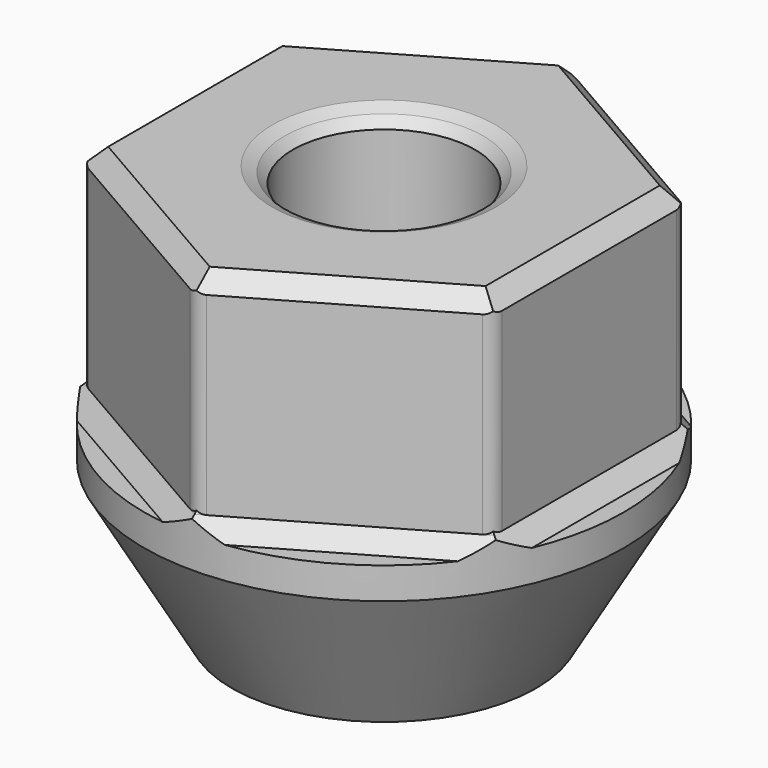
from build123d import *

# Parameters (mm, degrees)
F1_DEPTH       = 19
F2_D           = 8.4328
F2_CSINK_D     = 9.652
F2_CSINK_ANGLE = 82
F3_R           = 11.1125
F3_R_2         = 4.2164
F4_DEPTH       = 8.5
F5_SIZE2       = 7.039054482
F5_SIZE        = 4.064
F6_T1_DEPTH    = 14.8888999883
F6_T3_DEPTH    = 14.8888999883
F6_T5_DEPTH    = 14.8888999883
F6_T7_DEPTH    = 14.8888999883
F6_T9_DEPTH    = 14.8888999883
F7_T4_DEPTH    = 14.8888999883
F7_S5_R        = 11.1125
F7_T6_DEPTH    = 9
F7_T12_DEPTH   = 14.8888999883
F7_S13_R       = 11.1125
F7_T14_DEPTH   = 9
F7_T20_DEPTH   = 14.8888999883
F7_S21_R       = 11.1125
F7_T22_DEPTH   = 9
F7_T28_DEPTH   = 14.8888999883
F7_S29_R       = 11.1125
F7_T30_DEPTH   = 9
F7_T36_DEPTH   = 14.8888999883
F7_S37_R       = 11.1125
F7_T38_DEPTH   = 9
F7_T44_DEPTH   = 14.8888999883
F7_S45_R       = 11.1125
F7_T46_DEPTH   = 9
F7_T53_DEPTH   = 14.8888999883
F7_S54_R       = 11.1125
F7_T55_DEPTH   = 9
F7_T59_DEPTH   = 14.8888999883
F7_S60_R       = 11.1125
F7_T61_DEPTH   = 9
F7_T68_DEPTH   = 14.8888999883
F7_S69_R       = 11.1125
F7_T70_DEPTH   = 9
F7_T74_DEPTH   = 14.8888999883
F7_S75_R       = 11.1125
F7_T76_DEPTH   = 9
F7_T83_DEPTH   = 14.8888999883
F7_S84_R       = 11.1125
F7_T85_DEPTH   = 9
F7_T89_DEPTH   = 14.8888999883
F7_S90_R       = 11.1125
F7_T91_DEPTH   = 9
F7_T98_DEPTH   = 14.8888999883
F7_S99_R       = 11.1125
F7_T100_DEPTH  = 9
F7_T104_DEPTH  = 14.8888999883
F7_S105_R      = 11.1125
F7_T106_DEPTH  = 9
F7_T113_DEPTH  = 14.8888999883
F7_S114_R      = 11.1125
F7_T115_DEPTH  = 9
F7_T119_DEPTH  = 14.8888999883
F7_S120_R      = 11.1125
F7_T121_DEPTH  = 9
F7_T128_DEPTH  = 14.8888999883
F7_S129_R      = 11.1125
F7_T130_DEPTH  = 9
F7_T134_DEPTH  = 14.8888999883
F7_S135_R      = 11.1125
F7_T136_DEPTH  = 9
F8_T4_DEPTH    = 11.1757045256
F8_T10_DEPTH   = 11.1757045256
F8_T16_DEPTH   = 11.1757045256
F8_T22_DEPTH   = 11.1757045256
F8_T28_DEPTH   = 11.1757045256
F8_T34_DEPTH   = 11.1757045256
F8_T40_DEPTH   = 11.1757045256
F8_T46_DEPTH   = 11.1757045256
F8_T52_DEPTH   = 11.1757045256
F8_T58_DEPTH   = 11.1757045256
F8_T64_DEPTH   = 11.1757045256
F8_T70_DEPTH   = 11.1757045256
F8_T76_DEPTH   = 11.1757045256
F8_T82_DEPTH   = 11.1757045256
F8_T88_DEPTH   = 11.1757045256
F8_T94_DEPTH   = 11.1757045256
F8_T100_DEPTH  = 11.1757045256
F8_T106_DEPTH  = 11.1757045256


# Not quite as in the source:
# - a fillet or chamfer that OpenCascade refuses, or shapes differently, is made with other operations: its cross-section is extruded or revolved along the edge and cut away or added


with BuildPart() as f1:
    # F0 (on Top) → F1 (new body)
    with BuildSketch(Plane.XY):
        Polygon((9.5, -5.4848275573), (9.5, 5.4848275573), (0, 10.9696551146), (-9.5, 5.4848275573), (-9.5, -5.4848275573), (0, -10.9696551146), align=None)
    extrude(amount=-F1_DEPTH)

    # F2 (through all)
    with Locations(Plane.XY):
        with Locations((0, 0)):
            CounterSinkHole(F2_D / 2, F2_CSINK_D / 2, counter_sink_angle=F2_CSINK_ANGLE)

    # F3 (on face) → F4 (join)
    with BuildSketch(Plane(origin=(0, 0, -19), x_dir=(1, 0, 0), z_dir=(0, 0, -1))):
        Circle(F3_R)
        Circle(F3_R_2, mode=Mode.SUBTRACT)
    extrude(amount=-F4_DEPTH)

    # F5
    f5_edges = [f1.edges().sort_by_distance(p)[0] for p in [
        (-11.1125, 0, -19),
    ]]
    f5_side = f1.faces().sort_by_distance((-10.798191, 0, -19))[0]
    chamfer(f5_edges, length=F5_SIZE, length2=F5_SIZE2, reference=f5_side)

    # F6: chamfer of 0.762 on 7 edges, made by hand

    # F6_s2 → F6_t1 (cut)
    with BuildSketch(Plane.XZ.offset(-7.4444499941)):
        Polygon((9.5, -0.762), (8.738, 0), (9.5, 0), align=None)
        Polygon((-9.5, -0.762), (-8.738, 0), (-9.5, 0), align=None)
    extrude(amount=F6_T1_DEPTH, mode=Mode.SUBTRACT)

    # F6_s4 → F6_t3 (cut)
    with BuildSketch(Plane(origin=(-6.4470828121, -3.7222249971, 0), x_dir=(0, 0, 1), z_dir=(0.8660254038, 0.5, 0))):
        Polygon((-0.762, 9.5), (0, 8.738), (0, 9.5), align=None)
    extrude(amount=F6_T3_DEPTH, mode=Mode.SUBTRACT)

    # F6_s6 → F6_t5 (cut)
    with BuildSketch(Plane(origin=(6.4470828121, -3.7222249971, 0), x_dir=(0, 0, 1), z_dir=(-0.8660254038, 0.5, 0))):
        Polygon((-0.762, 9.5), (0, 8.738), (0, 9.5), align=None)
    extrude(amount=F6_T5_DEPTH, mode=Mode.SUBTRACT)

    # F6_s8 → F6_t7 (cut)
    with BuildSketch(Plane(origin=(-6.4470828121, 3.7222249971, 0), x_dir=(0, 0, 1), z_dir=(0.8660254038, -0.5, 0))):
        Polygon((-0.762, 9.5), (0, 8.738), (0, 9.5), align=None)
    extrude(amount=F6_T7_DEPTH, mode=Mode.SUBTRACT)

    # F6_s10 → F6_t9 (cut)
    with BuildSketch(Plane(origin=(6.4470828121, 3.7222249971, 0), x_dir=(0, 0, 1), z_dir=(-0.8660254038, -0.5, 0))):
        Polygon((-0.762, 9.5), (0, 8.738), (0, 9.5), align=None)
    extrude(amount=F6_T9_DEPTH, mode=Mode.SUBTRACT)

    # F6_s11 → F6_t12 (revolve, cut)
    with BuildSketch(Plane.XZ):
        Polygon((5.1727200241, 0), (4.5972787828, -0.2624888611), (4.8251319511, 0), align=None)
    revolve(axis=Axis((0, 0, 0), (0, 0, 1)), mode=Mode.SUBTRACT)

    # F7: chamfer of 0.762 on 6 edges, made by hand


with BuildPart() as f7_tool2:
    # F7_s3 → F7_t4 (new body)
    with BuildSketch(Plane(origin=(-6.4470828121, 3.7222249971, 0), x_dir=(0, 0, 1), z_dir=(0.8660254038, -0.5, 0))):
        Polygon((-10.5, 10.262), (-9.738, 9.5), (-10.5, 9.5), align=None)
    extrude(amount=F7_T4_DEPTH)

    # F7_s5 → F7_t6 (intersect, symmetric)
    with BuildSketch(Plane.XY.offset(-10.1)):
        Circle(F7_S5_R)
    extrude(amount=F7_T6_DEPTH, both=True, mode=Mode.INTERSECT)

    split(bisect_by=Plane(origin=(4.75, -8.227241336, 0), x_dir=(0, 0, 1), z_dir=(-0.5, 0.8660254038, 0)), keep=Keep.TOP)

    split(bisect_by=Plane.YZ.offset(-9.5), keep=Keep.TOP)


with BuildPart() as f1_1:
    add(f1.part)

    # F7_t1: union F7_tool2
    add(f7_tool2.part)


with BuildPart() as f7_tool10:
    # F7_s11 → F7_t12 (new body)
    with BuildSketch(Plane(origin=(-6.4470828121, -3.7222249971, 0), x_dir=(0, 0, 1), z_dir=(0.8660254038, 0.5, 0))):
        Polygon((-10.5, 10.262), (-9.738, 9.5), (-10.5, 9.5), align=None)
    extrude(amount=F7_T12_DEPTH)

    # F7_s13 → F7_t14 (intersect, symmetric)
    with BuildSketch(Plane.XY.offset(-10.1)):
        Circle(F7_S13_R)
    extrude(amount=F7_T14_DEPTH, both=True, mode=Mode.INTERSECT)

    split(bisect_by=Plane.YZ.offset(9.5), keep=Keep.BOTTOM)

    split(bisect_by=Plane(origin=(-4.75, -8.227241336, 0), x_dir=(0, 0, 1), z_dir=(0.5, 0.8660254038, 0)), keep=Keep.TOP)


with BuildPart() as f1_2:
    add(f1_1.part)

    # F7_t9: union F7_tool10
    add(f7_tool10.part)


with BuildPart() as f7_tool18:
    # F7_s19 → F7_t20 (new body)
    with BuildSketch(Plane.XZ.offset(7.4444499941)):
        Polygon((10.262, -10.5), (9.5, -9.738), (9.5, -10.5), align=None)
    extrude(amount=-F7_T20_DEPTH)

    # F7_s21 → F7_t22 (intersect, symmetric)
    with BuildSketch(Plane.XY.offset(-10.1)):
        Circle(F7_S21_R)
    extrude(amount=F7_T22_DEPTH, both=True, mode=Mode.INTERSECT)

    split(bisect_by=Plane(origin=(4.75, -8.227241336, 0), x_dir=(0, 0, 1), z_dir=(-0.5, 0.8660254038, 0)), keep=Keep.TOP)

    split(bisect_by=Plane(origin=(4.75, 8.227241336, 0), x_dir=(0, 0, 1), z_dir=(-0.5, -0.8660254038, 0)), keep=Keep.TOP)


with BuildPart() as f1_3:
    add(f1_2.part)

    # F7_t17: union F7_tool18
    add(f7_tool18.part)


with BuildPart() as f7_tool26:
    # F7_s27 → F7_t28 (new body)
    with BuildSketch(Plane(origin=(6.4470828121, -3.7222249971, 0), x_dir=(0, 0, 1), z_dir=(-0.8660254038, 0.5, 0))):
        Polygon((-10.5, 10.262), (-9.738, 9.5), (-10.5, 9.5), align=None)
    extrude(amount=F7_T28_DEPTH)

    # F7_s29 → F7_t30 (intersect, symmetric)
    with BuildSketch(Plane.XY.offset(-10.1)):
        Circle(F7_S29_R)
    extrude(amount=F7_T30_DEPTH, both=True, mode=Mode.INTERSECT)

    split(bisect_by=Plane(origin=(-4.75, 8.227241336, 0), x_dir=(0, 0, 1), z_dir=(0.5, -0.8660254038, 0)), keep=Keep.TOP)

    split(bisect_by=Plane.YZ.offset(9.5), keep=Keep.BOTTOM)


with BuildPart() as f1_4:
    add(f1_3.part)

    # F7_t25: union F7_tool26
    add(f7_tool26.part)


with BuildPart() as f7_tool34:
    # F7_s35 → F7_t36 (new body)
    with BuildSketch(Plane(origin=(6.4470828121, 3.7222249971, 0), x_dir=(0, 0, 1), z_dir=(-0.8660254038, -0.5, 0))):
        Polygon((-10.5, 10.262), (-9.738, 9.5), (-10.5, 9.5), align=None)
    extrude(amount=F7_T36_DEPTH)

    # F7_s37 → F7_t38 (intersect, symmetric)
    with BuildSketch(Plane.XY.offset(-10.1)):
        Circle(F7_S37_R)
    extrude(amount=F7_T38_DEPTH, both=True, mode=Mode.INTERSECT)

    split(bisect_by=Plane.YZ.offset(-9.5), keep=Keep.TOP)

    split(bisect_by=Plane(origin=(4.75, 8.227241336, 0), x_dir=(0, 0, 1), z_dir=(-0.5, -0.8660254038, 0)), keep=Keep.TOP)


with BuildPart() as f1_5:
    add(f1_4.part)

    # F7_t33: union F7_tool34
    add(f7_tool34.part)


with BuildPart() as f7_tool42:
    # F7_s43 → F7_t44 (new body)
    with BuildSketch(Plane.XZ.offset(-7.4444499941)):
        Polygon((-10.262, -10.5), (-9.5, -9.738), (-9.5, -10.5), align=None)
    extrude(amount=F7_T44_DEPTH)

    # F7_s45 → F7_t46 (intersect, symmetric)
    with BuildSketch(Plane.XY.offset(-10.1)):
        Circle(F7_S45_R)
    extrude(amount=F7_T46_DEPTH, both=True, mode=Mode.INTERSECT)

    split(bisect_by=Plane(origin=(-4.75, -8.227241336, 0), x_dir=(0, 0, 1), z_dir=(0.5, 0.8660254038, 0)), keep=Keep.TOP)

    split(bisect_by=Plane(origin=(-4.75, 8.227241336, 0), x_dir=(0, 0, 1), z_dir=(0.5, -0.8660254038, 0)), keep=Keep.TOP)


with BuildPart() as f1_6:
    add(f1_5.part)

    # F7_t41: union F7_tool42
    add(f7_tool42.part)


with BuildPart() as f7_tool51:
    # F7_s52 → F7_t53 (new body)
    with BuildSketch(Plane(origin=(-6.4470828121, 3.7222249971, 0), x_dir=(0, 0, 1), z_dir=(0.8660254038, -0.5, 0))):
        Polygon((-10.5, 10.262), (-9.738, 9.5), (-10.5, 9.5), align=None)
    extrude(amount=F7_T53_DEPTH)

    # F7_s54 → F7_t55 (intersect, symmetric)
    with BuildSketch(Plane.XY.offset(-10.1)):
        Circle(F7_S54_R)
    extrude(amount=F7_T55_DEPTH, both=True, mode=Mode.INTERSECT)

    split(bisect_by=Plane.YZ.offset(-9.5), keep=Keep.BOTTOM)


with BuildPart() as f7_tool57:
    # F7_s58 → F7_t59 (new body)
    with BuildSketch(Plane.XZ.offset(-7.4444499941)):
        Polygon((-10.262, -10.5), (-9.5, -9.738), (-9.5, -10.5), align=None)
    extrude(amount=F7_T59_DEPTH)

    # F7_s60 → F7_t61 (intersect, symmetric)
    with BuildSketch(Plane.XY.offset(-10.1)):
        Circle(F7_S60_R)
    extrude(amount=F7_T61_DEPTH, both=True, mode=Mode.INTERSECT)

    split(bisect_by=Plane(origin=(-4.75, -8.227241336, 0), x_dir=(0, 0, 1), z_dir=(-0.5, -0.8660254038, 0)), keep=Keep.TOP)


with BuildPart() as f7_tool51_1:
    add(f7_tool51.part)

    # F7_t63: intersect F7_tool57
    add(f7_tool57.part, mode=Mode.INTERSECT)


with BuildPart() as f1_7:
    add(f1_6.part)

    # F7_t49: union F7_tool51
    add(f7_tool51_1.part)


with BuildPart() as f7_tool66:
    # F7_s67 → F7_t68 (new body)
    with BuildSketch(Plane(origin=(-6.4470828121, -3.7222249971, 0), x_dir=(0, 0, 1), z_dir=(0.8660254038, 0.5, 0))):
        Polygon((-10.5, 10.262), (-9.738, 9.5), (-10.5, 9.5), align=None)
    extrude(amount=F7_T68_DEPTH)

    # F7_s69 → F7_t70 (intersect, symmetric)
    with BuildSketch(Plane.XY.offset(-10.1)):
        Circle(F7_S69_R)
    extrude(amount=F7_T70_DEPTH, both=True, mode=Mode.INTERSECT)

    split(bisect_by=Plane(origin=(-4.75, -8.227241336, 0), x_dir=(0, 0, 1), z_dir=(-0.5, -0.8660254038, 0)), keep=Keep.TOP)


with BuildPart() as f7_tool72:
    # F7_s73 → F7_t74 (new body)
    with BuildSketch(Plane(origin=(-6.4470828121, 3.7222249971, 0), x_dir=(0, 0, 1), z_dir=(0.8660254038, -0.5, 0))):
        Polygon((-10.5, 10.262), (-9.738, 9.5), (-10.5, 9.5), align=None)
    extrude(amount=F7_T74_DEPTH)

    # F7_s75 → F7_t76 (intersect, symmetric)
    with BuildSketch(Plane.XY.offset(-10.1)):
        Circle(F7_S75_R)
    extrude(amount=F7_T76_DEPTH, both=True, mode=Mode.INTERSECT)

    split(bisect_by=Plane(origin=(4.75, -8.227241336, 0), x_dir=(0, 0, 1), z_dir=(0.5, -0.8660254038, 0)), keep=Keep.TOP)


with BuildPart() as f7_tool66_1:
    add(f7_tool66.part)

    # F7_t78: intersect F7_tool72
    add(f7_tool72.part, mode=Mode.INTERSECT)


with BuildPart() as f1_8:
    add(f1_7.part)

    # F7_t64: union F7_tool66
    add(f7_tool66_1.part)


with BuildPart() as f7_tool81:
    # F7_s82 → F7_t83 (new body)
    with BuildSketch(Plane(origin=(-6.4470828121, -3.7222249971, 0), x_dir=(0, 0, 1), z_dir=(0.8660254038, 0.5, 0))):
        Polygon((-10.5, 10.262), (-9.738, 9.5), (-10.5, 9.5), align=None)
    extrude(amount=F7_T83_DEPTH)

    # F7_s84 → F7_t85 (intersect, symmetric)
    with BuildSketch(Plane.XY.offset(-10.1)):
        Circle(F7_S84_R)
    extrude(amount=F7_T85_DEPTH, both=True, mode=Mode.INTERSECT)

    split(bisect_by=Plane.YZ.offset(9.5), keep=Keep.TOP)


with BuildPart() as f7_tool87:
    # F7_s88 → F7_t89 (new body)
    with BuildSketch(Plane.XZ.offset(7.4444499941)):
        Polygon((10.262, -10.5), (9.5, -9.738), (9.5, -10.5), align=None)
    extrude(amount=-F7_T89_DEPTH)

    # F7_s90 → F7_t91 (intersect, symmetric)
    with BuildSketch(Plane.XY.offset(-10.1)):
        Circle(F7_S90_R)
    extrude(amount=F7_T91_DEPTH, both=True, mode=Mode.INTERSECT)

    split(bisect_by=Plane(origin=(4.75, -8.227241336, 0), x_dir=(0, 0, 1), z_dir=(0.5, -0.8660254038, 0)), keep=Keep.TOP)


with BuildPart() as f7_tool81_1:
    add(f7_tool81.part)

    # F7_t93: intersect F7_tool87
    add(f7_tool87.part, mode=Mode.INTERSECT)


with BuildPart() as f1_9:
    add(f1_8.part)

    # F7_t79: union F7_tool81
    add(f7_tool81_1.part)


with BuildPart() as f7_tool96:
    # F7_s97 → F7_t98 (new body)
    with BuildSketch(Plane(origin=(6.4470828121, -3.7222249971, 0), x_dir=(0, 0, 1), z_dir=(-0.8660254038, 0.5, 0))):
        Polygon((-10.5, 10.262), (-9.738, 9.5), (-10.5, 9.5), align=None)
    extrude(amount=F7_T98_DEPTH)

    # F7_s99 → F7_t100 (intersect, symmetric)
    with BuildSketch(Plane.XY.offset(-10.1)):
        Circle(F7_S99_R)
    extrude(amount=F7_T100_DEPTH, both=True, mode=Mode.INTERSECT)

    split(bisect_by=Plane.YZ.offset(9.5), keep=Keep.TOP)


with BuildPart() as f7_tool102:
    # F7_s103 → F7_t104 (new body)
    with BuildSketch(Plane.XZ.offset(7.4444499941)):
        Polygon((10.262, -10.5), (9.5, -9.738), (9.5, -10.5), align=None)
    extrude(amount=-F7_T104_DEPTH)

    # F7_s105 → F7_t106 (intersect, symmetric)
    with BuildSketch(Plane.XY.offset(-10.1)):
        Circle(F7_S105_R)
    extrude(amount=F7_T106_DEPTH, both=True, mode=Mode.INTERSECT)

    split(bisect_by=Plane(origin=(4.75, 8.227241336, 0), x_dir=(0, 0, 1), z_dir=(0.5, 0.8660254038, 0)), keep=Keep.TOP)


with BuildPart() as f7_tool96_1:
    add(f7_tool96.part)

    # F7_t108: intersect F7_tool102
    add(f7_tool102.part, mode=Mode.INTERSECT)


with BuildPart() as f1_10:
    add(f1_9.part)

    # F7_t94: union F7_tool96
    add(f7_tool96_1.part)


with BuildPart() as f7_tool111:
    # F7_s112 → F7_t113 (new body)
    with BuildSketch(Plane(origin=(6.4470828121, 3.7222249971, 0), x_dir=(0, 0, 1), z_dir=(-0.8660254038, -0.5, 0))):
        Polygon((-10.5, 10.262), (-9.738, 9.5), (-10.5, 9.5), align=None)
    extrude(amount=F7_T113_DEPTH)

    # F7_s114 → F7_t115 (intersect, symmetric)
    with BuildSketch(Plane.XY.offset(-10.1)):
        Circle(F7_S114_R)
    extrude(amount=F7_T115_DEPTH, both=True, mode=Mode.INTERSECT)

    split(bisect_by=Plane(origin=(4.75, 8.227241336, 0), x_dir=(0, 0, 1), z_dir=(0.5, 0.8660254038, 0)), keep=Keep.TOP)


with BuildPart() as f7_tool117:
    # F7_s118 → F7_t119 (new body)
    with BuildSketch(Plane(origin=(6.4470828121, -3.7222249971, 0), x_dir=(0, 0, 1), z_dir=(-0.8660254038, 0.5, 0))):
        Polygon((-10.5, 10.262), (-9.738, 9.5), (-10.5, 9.5), align=None)
    extrude(amount=F7_T119_DEPTH)

    # F7_s120 → F7_t121 (intersect, symmetric)
    with BuildSketch(Plane.XY.offset(-10.1)):
        Circle(F7_S120_R)
    extrude(amount=F7_T121_DEPTH, both=True, mode=Mode.INTERSECT)

    split(bisect_by=Plane(origin=(-4.75, 8.227241336, 0), x_dir=(0, 0, 1), z_dir=(-0.5, 0.8660254038, 0)), keep=Keep.TOP)


with BuildPart() as f7_tool111_1:
    add(f7_tool111.part)

    # F7_t123: intersect F7_tool117
    add(f7_tool117.part, mode=Mode.INTERSECT)


with BuildPart() as f1_11:
    add(f1_10.part)

    # F7_t109: union F7_tool111
    add(f7_tool111_1.part)


with BuildPart() as f7_tool126:
    # F7_s127 → F7_t128 (new body)
    with BuildSketch(Plane.XZ.offset(-7.4444499941)):
        Polygon((-10.262, -10.5), (-9.5, -9.738), (-9.5, -10.5), align=None)
    extrude(amount=F7_T128_DEPTH)

    # F7_s129 → F7_t130 (intersect, symmetric)
    with BuildSketch(Plane.XY.offset(-10.1)):
        Circle(F7_S129_R)
    extrude(amount=F7_T130_DEPTH, both=True, mode=Mode.INTERSECT)

    split(bisect_by=Plane(origin=(-4.75, 8.227241336, 0), x_dir=(0, 0, 1), z_dir=(-0.5, 0.8660254038, 0)), keep=Keep.TOP)


with BuildPart() as f7_tool132:
    # F7_s133 → F7_t134 (new body)
    with BuildSketch(Plane(origin=(6.4470828121, 3.7222249971, 0), x_dir=(0, 0, 1), z_dir=(-0.8660254038, -0.5, 0))):
        Polygon((-10.5, 10.262), (-9.738, 9.5), (-10.5, 9.5), align=None)
    extrude(amount=F7_T134_DEPTH)

    # F7_s135 → F7_t136 (intersect, symmetric)
    with BuildSketch(Plane.XY.offset(-10.1)):
        Circle(F7_S135_R)
    extrude(amount=F7_T136_DEPTH, both=True, mode=Mode.INTERSECT)

    split(bisect_by=Plane.YZ.offset(-9.5), keep=Keep.BOTTOM)


with BuildPart() as f7_tool126_1:
    add(f7_tool126.part)

    # F7_t138: intersect F7_tool132
    add(f7_tool132.part, mode=Mode.INTERSECT)


with BuildPart() as f1_12:
    add(f1_11.part)

    # F7_t124: union F7_tool126
    add(f7_tool126_1.part)

    # F8: fillet of radius 0.762 on 6 edges, made by hand


with BuildPart() as f8_tool2:
    # F8_s3 → F8_t4 (new body)
    with BuildSketch(Plane.XY.offset(0.3378522628)):
        with BuildLine():
            ThreePointArc((9.5, -5.0448866522), (9.3979113577, -5.4258866522), (9.119, -5.7047980099))
            Line((9.119, -5.7047980099), (9.5, -5.4848275573))
            Line((9.5, -5.4848275573), (9.5, -5.0448866522))
        make_face()
    extrude(amount=-F8_T4_DEPTH)

    split(bisect_by=Plane(origin=(-0.119, 0, -0.119), x_dir=(0, 1, 0), z_dir=(0.7071067812, 0, 0.7071067812)), keep=Keep.TOP)

    split(bisect_by=Plane(origin=(-0.0595, 0.1030570231, -0.119), x_dir=(0.8660254038, 0.5, 0), z_dir=(0.3535533906, -0.6123724357, 0.7071067812)), keep=Keep.TOP)


with BuildPart() as f1_13:
    add(f1_12.part)

    # F8_t1: cut F8_tool2
    add(f8_tool2.part, mode=Mode.SUBTRACT)


with BuildPart() as f8_tool8:
    # F8_s9 → F8_t10 (new body)
    with BuildSketch(Plane.XY.offset(0.3378522628)):
        with BuildLine():
            ThreePointArc((9.5, -5.0448866522), (9.3979113577, -5.4258866522), (9.119, -5.7047980099))
            Line((9.119, -5.7047980099), (9.5, -5.4848275573))
            Line((9.5, -5.4848275573), (9.5, -5.0448866522))
        make_face()
    extrude(amount=-F8_T10_DEPTH)

    split(bisect_by=Plane(origin=(-0.119, 0, -0.119), x_dir=(0, 1, 0), z_dir=(-0.7071067812, 0, -0.7071067812)), keep=Keep.TOP)

    split(bisect_by=Plane(origin=(-0.0595, 0.1030570231, -0.119), x_dir=(0.8660254038, 0.5, 0), z_dir=(0.3535533906, -0.6123724357, 0.7071067812)), keep=Keep.TOP)


with BuildPart() as f1_14:
    add(f1_13.part)

    # F8_t7: cut F8_tool8
    add(f8_tool8.part, mode=Mode.SUBTRACT)


with BuildPart() as f8_tool14:
    # F8_s15 → F8_t16 (new body)
    with BuildSketch(Plane.XY.offset(0.3378522628)):
        with BuildLine():
            ThreePointArc((9.5, -5.0448866522), (9.3979113577, -5.4258866522), (9.119, -5.7047980099))
            Line((9.119, -5.7047980099), (9.5, -5.4848275573))
            Line((9.5, -5.4848275573), (9.5, -5.0448866522))
        make_face()
    extrude(amount=-F8_T16_DEPTH)

    split(bisect_by=Plane(origin=(-0.119, 0, -0.119), x_dir=(0, 1, 0), z_dir=(0.7071067812, 0, 0.7071067812)), keep=Keep.TOP)

    split(bisect_by=Plane(origin=(-0.0595, 0.1030570231, -0.119), x_dir=(-0.8660254038, -0.5, 0), z_dir=(-0.3535533906, 0.6123724357, -0.7071067812)), keep=Keep.TOP)


with BuildPart() as f1_15:
    add(f1_14.part)

    # F8_t13: cut F8_tool14
    add(f8_tool14.part, mode=Mode.SUBTRACT)


with BuildPart() as f8_tool20:
    # F8_s21 → F8_t22 (new body)
    with BuildSketch(Plane.XY.offset(0.3378522628)):
        with BuildLine():
            ThreePointArc((-0.381, -10.749684662), (0, -10.8517733044), (0.381, -10.749684662))
            Line((0.381, -10.749684662), (0, -10.9696551146))
            Line((0, -10.9696551146), (-0.381, -10.749684662))
        make_face()
    extrude(amount=-F8_T22_DEPTH)

    split(bisect_by=Plane(origin=(0.0595, 0.1030570231, -0.119), x_dir=(0.8660254038, -0.5, 0), z_dir=(-0.3535533906, -0.6123724357, 0.7071067812)), keep=Keep.TOP)

    split(bisect_by=Plane(origin=(-0.0595, 0.1030570231, -0.119), x_dir=(0.8660254038, 0.5, 0), z_dir=(0.3535533906, -0.6123724357, 0.7071067812)), keep=Keep.TOP)


with BuildPart() as f1_16:
    add(f1_15.part)

    # F8_t19: cut F8_tool20
    add(f8_tool20.part, mode=Mode.SUBTRACT)


with BuildPart() as f8_tool26:
    # F8_s27 → F8_t28 (new body)
    with BuildSketch(Plane.XY.offset(0.3378522628)):
        with BuildLine():
            ThreePointArc((-0.381, -10.749684662), (0, -10.8517733044), (0.381, -10.749684662))
            Line((0.381, -10.749684662), (0, -10.9696551146))
            Line((0, -10.9696551146), (-0.381, -10.749684662))
        make_face()
    extrude(amount=-F8_T28_DEPTH)

    split(bisect_by=Plane(origin=(0.0595, 0.1030570231, -0.119), x_dir=(-0.8660254038, 0.5, 0), z_dir=(0.3535533906, 0.6123724357, -0.7071067812)), keep=Keep.TOP)

    split(bisect_by=Plane(origin=(-0.0595, 0.1030570231, -0.119), x_dir=(0.8660254038, 0.5, 0), z_dir=(0.3535533906, -0.6123724357, 0.7071067812)), keep=Keep.TOP)


with BuildPart() as f1_17:
    add(f1_16.part)

    # F8_t25: cut F8_tool26
    add(f8_tool26.part, mode=Mode.SUBTRACT)


with BuildPart() as f8_tool32:
    # F8_s33 → F8_t34 (new body)
    with BuildSketch(Plane.XY.offset(0.3378522628)):
        with BuildLine():
            ThreePointArc((-0.381, -10.749684662), (0, -10.8517733044), (0.381, -10.749684662))
            Line((0.381, -10.749684662), (0, -10.9696551146))
            Line((0, -10.9696551146), (-0.381, -10.749684662))
        make_face()
    extrude(amount=-F8_T34_DEPTH)

    split(bisect_by=Plane(origin=(0.0595, 0.1030570231, -0.119), x_dir=(0.8660254038, -0.5, 0), z_dir=(-0.3535533906, -0.6123724357, 0.7071067812)), keep=Keep.TOP)

    split(bisect_by=Plane(origin=(-0.0595, 0.1030570231, -0.119), x_dir=(-0.8660254038, -0.5, 0), z_dir=(-0.3535533906, 0.6123724357, -0.7071067812)), keep=Keep.TOP)


with BuildPart() as f1_18:
    add(f1_17.part)

    # F8_t31: cut F8_tool32
    add(f8_tool32.part, mode=Mode.SUBTRACT)


with BuildPart() as f8_tool38:
    # F8_s39 → F8_t40 (new body)
    with BuildSketch(Plane.XY.offset(0.3378522628)):
        with BuildLine():
            ThreePointArc((-9.5, -5.0448866522), (-9.3979113577, -5.4258866522), (-9.119, -5.7047980099))
            Line((-9.119, -5.7047980099), (-9.5, -5.4848275573))
            Line((-9.5, -5.4848275573), (-9.5, -5.0448866522))
        make_face()
    extrude(amount=-F8_T40_DEPTH)

    split(bisect_by=Plane(origin=(0.119, 0, -0.119), x_dir=(0, 1, 0), z_dir=(-0.7071067812, 0, 0.7071067812)), keep=Keep.TOP)

    split(bisect_by=Plane(origin=(0.0595, 0.1030570231, -0.119), x_dir=(0.8660254038, -0.5, 0), z_dir=(-0.3535533906, -0.6123724357, 0.7071067812)), keep=Keep.TOP)


with BuildPart() as f1_19:
    add(f1_18.part)

    # F8_t37: cut F8_tool38
    add(f8_tool38.part, mode=Mode.SUBTRACT)


with BuildPart() as f8_tool44:
    # F8_s45 → F8_t46 (new body)
    with BuildSketch(Plane.XY.offset(0.3378522628)):
        with BuildLine():
            ThreePointArc((-9.5, -5.0448866522), (-9.3979113577, -5.4258866522), (-9.119, -5.7047980099))
            Line((-9.119, -5.7047980099), (-9.5, -5.4848275573))
            Line((-9.5, -5.4848275573), (-9.5, -5.0448866522))
        make_face()
    extrude(amount=-F8_T46_DEPTH)

    split(bisect_by=Plane(origin=(0.119, 0, -0.119), x_dir=(0, 1, 0), z_dir=(0.7071067812, 0, -0.7071067812)), keep=Keep.TOP)

    split(bisect_by=Plane(origin=(0.0595, 0.1030570231, -0.119), x_dir=(0.8660254038, -0.5, 0), z_dir=(-0.3535533906, -0.6123724357, 0.7071067812)), keep=Keep.TOP)


with BuildPart() as f1_20:
    add(f1_19.part)

    # F8_t43: cut F8_tool44
    add(f8_tool44.part, mode=Mode.SUBTRACT)


with BuildPart() as f8_tool50:
    # F8_s51 → F8_t52 (new body)
    with BuildSketch(Plane.XY.offset(0.3378522628)):
        with BuildLine():
            ThreePointArc((-9.5, -5.0448866522), (-9.3979113577, -5.4258866522), (-9.119, -5.7047980099))
            Line((-9.119, -5.7047980099), (-9.5, -5.4848275573))
            Line((-9.5, -5.4848275573), (-9.5, -5.0448866522))
        make_face()
    extrude(amount=-F8_T52_DEPTH)

    split(bisect_by=Plane(origin=(0.119, 0, -0.119), x_dir=(0, 1, 0), z_dir=(-0.7071067812, 0, 0.7071067812)), keep=Keep.TOP)

    split(bisect_by=Plane(origin=(0.0595, 0.1030570231, -0.119), x_dir=(-0.8660254038, 0.5, 0), z_dir=(0.3535533906, 0.6123724357, -0.7071067812)), keep=Keep.TOP)


with BuildPart() as f1_21:
    add(f1_20.part)

    # F8_t49: cut F8_tool50
    add(f8_tool50.part, mode=Mode.SUBTRACT)


with BuildPart() as f8_tool56:
    # F8_s57 → F8_t58 (new body)
    with BuildSketch(Plane.XY.offset(0.3378522628)):
        with BuildLine():
            ThreePointArc((-9.119, 5.7047980099), (-9.3979113577, 5.4258866522), (-9.5, 5.0448866522))
            Line((-9.5, 5.0448866522), (-9.5, 5.4848275573))
            Line((-9.5, 5.4848275573), (-9.119, 5.7047980099))
        make_face()
    extrude(amount=-F8_T58_DEPTH)

    split(bisect_by=Plane(origin=(0.0595, -0.1030570231, -0.119), x_dir=(-0.8660254038, -0.5, 0), z_dir=(-0.3535533906, 0.6123724357, 0.7071067812)), keep=Keep.TOP)

    split(bisect_by=Plane(origin=(0.119, 0, -0.119), x_dir=(0, 1, 0), z_dir=(-0.7071067812, 0, 0.7071067812)), keep=Keep.TOP)


with BuildPart() as f1_22:
    add(f1_21.part)

    # F8_t55: cut F8_tool56
    add(f8_tool56.part, mode=Mode.SUBTRACT)


with BuildPart() as f8_tool62:
    # F8_s63 → F8_t64 (new body)
    with BuildSketch(Plane.XY.offset(0.3378522628)):
        with BuildLine():
            ThreePointArc((-9.119, 5.7047980099), (-9.3979113577, 5.4258866522), (-9.5, 5.0448866522))
            Line((-9.5, 5.0448866522), (-9.5, 5.4848275573))
            Line((-9.5, 5.4848275573), (-9.119, 5.7047980099))
        make_face()
    extrude(amount=-F8_T64_DEPTH)

    split(bisect_by=Plane(origin=(0.0595, -0.1030570231, -0.119), x_dir=(0.8660254038, 0.5, 0), z_dir=(0.3535533906, -0.6123724357, -0.7071067812)), keep=Keep.TOP)

    split(bisect_by=Plane(origin=(0.119, 0, -0.119), x_dir=(0, 1, 0), z_dir=(-0.7071067812, 0, 0.7071067812)), keep=Keep.TOP)


with BuildPart() as f1_23:
    add(f1_22.part)

    # F8_t61: cut F8_tool62
    add(f8_tool62.part, mode=Mode.SUBTRACT)


with BuildPart() as f8_tool68:
    # F8_s69 → F8_t70 (new body)
    with BuildSketch(Plane.XY.offset(0.3378522628)):
        with BuildLine():
            ThreePointArc((-9.119, 5.7047980099), (-9.3979113577, 5.4258866522), (-9.5, 5.0448866522))
            Line((-9.5, 5.0448866522), (-9.5, 5.4848275573))
            Line((-9.5, 5.4848275573), (-9.119, 5.7047980099))
        make_face()
    extrude(amount=-F8_T70_DEPTH)

    split(bisect_by=Plane(origin=(0.0595, -0.1030570231, -0.119), x_dir=(-0.8660254038, -0.5, 0), z_dir=(-0.3535533906, 0.6123724357, 0.7071067812)), keep=Keep.TOP)

    split(bisect_by=Plane(origin=(0.119, 0, -0.119), x_dir=(0, 1, 0), z_dir=(0.7071067812, 0, -0.7071067812)), keep=Keep.TOP)


with BuildPart() as f1_24:
    add(f1_23.part)

    # F8_t67: cut F8_tool68
    add(f8_tool68.part, mode=Mode.SUBTRACT)


with BuildPart() as f8_tool74:
    # F8_s75 → F8_t76 (new body)
    with BuildSketch(Plane.XY.offset(0.3378522628)):
        with BuildLine():
            ThreePointArc((0.381, 10.749684662), (0, 10.8517733044), (-0.381, 10.749684662))
            Line((-0.381, 10.749684662), (0, 10.9696551146))
            Line((0, 10.9696551146), (0.381, 10.749684662))
        make_face()
    extrude(amount=-F8_T76_DEPTH)

    split(bisect_by=Plane(origin=(-0.0595, -0.1030570231, -0.119), x_dir=(-0.8660254038, 0.5, 0), z_dir=(0.3535533906, 0.6123724357, 0.7071067812)), keep=Keep.TOP)

    split(bisect_by=Plane(origin=(0.0595, -0.1030570231, -0.119), x_dir=(-0.8660254038, -0.5, 0), z_dir=(-0.3535533906, 0.6123724357, 0.7071067812)), keep=Keep.TOP)


with BuildPart() as f1_25:
    add(f1_24.part)

    # F8_t73: cut F8_tool74
    add(f8_tool74.part, mode=Mode.SUBTRACT)


with BuildPart() as f8_tool80:
    # F8_s81 → F8_t82 (new body)
    with BuildSketch(Plane.XY.offset(0.3378522628)):
        with BuildLine():
            ThreePointArc((0.381, 10.749684662), (0, 10.8517733044), (-0.381, 10.749684662))
            Line((-0.381, 10.749684662), (0, 10.9696551146))
            Line((0, 10.9696551146), (0.381, 10.749684662))
        make_face()
    extrude(amount=-F8_T82_DEPTH)

    split(bisect_by=Plane(origin=(-0.0595, -0.1030570231, -0.119), x_dir=(0.8660254038, -0.5, 0), z_dir=(-0.3535533906, -0.6123724357, -0.7071067812)), keep=Keep.TOP)

    split(bisect_by=Plane(origin=(0.0595, -0.1030570231, -0.119), x_dir=(-0.8660254038, -0.5, 0), z_dir=(-0.3535533906, 0.6123724357, 0.7071067812)), keep=Keep.TOP)


with BuildPart() as f1_26:
    add(f1_25.part)

    # F8_t79: cut F8_tool80
    add(f8_tool80.part, mode=Mode.SUBTRACT)


with BuildPart() as f8_tool86:
    # F8_s87 → F8_t88 (new body)
    with BuildSketch(Plane.XY.offset(0.3378522628)):
        with BuildLine():
            ThreePointArc((0.381, 10.749684662), (0, 10.8517733044), (-0.381, 10.749684662))
            Line((-0.381, 10.749684662), (0, 10.9696551146))
            Line((0, 10.9696551146), (0.381, 10.749684662))
        make_face()
    extrude(amount=-F8_T88_DEPTH)

    split(bisect_by=Plane(origin=(-0.0595, -0.1030570231, -0.119), x_dir=(-0.8660254038, 0.5, 0), z_dir=(0.3535533906, 0.6123724357, 0.7071067812)), keep=Keep.TOP)

    split(bisect_by=Plane(origin=(0.0595, -0.1030570231, -0.119), x_dir=(0.8660254038, 0.5, 0), z_dir=(0.3535533906, -0.6123724357, -0.7071067812)), keep=Keep.TOP)


with BuildPart() as f1_27:
    add(f1_26.part)

    # F8_t85: cut F8_tool86
    add(f8_tool86.part, mode=Mode.SUBTRACT)


with BuildPart() as f8_tool92:
    # F8_s93 → F8_t94 (new body)
    with BuildSketch(Plane.XY.offset(0.3378522628)):
        with BuildLine():
            ThreePointArc((9.5, 5.0448866522), (9.3979113577, 5.4258866522), (9.119, 5.7047980099))
            Line((9.119, 5.7047980099), (9.5, 5.4848275573))
            Line((9.5, 5.4848275573), (9.5, 5.0448866522))
        make_face()
    extrude(amount=-F8_T94_DEPTH)

    split(bisect_by=Plane(origin=(-0.119, 0, -0.119), x_dir=(0, 1, 0), z_dir=(0.7071067812, 0, 0.7071067812)), keep=Keep.TOP)

    split(bisect_by=Plane(origin=(-0.0595, -0.1030570231, -0.119), x_dir=(-0.8660254038, 0.5, 0), z_dir=(0.3535533906, 0.6123724357, 0.7071067812)), keep=Keep.TOP)


with BuildPart() as f1_28:
    add(f1_27.part)

    # F8_t91: cut F8_tool92
    add(f8_tool92.part, mode=Mode.SUBTRACT)


with BuildPart() as f8_tool98:
    # F8_s99 → F8_t100 (new body)
    with BuildSketch(Plane.XY.offset(0.3378522628)):
        with BuildLine():
            ThreePointArc((9.5, 5.0448866522), (9.3979113577, 5.4258866522), (9.119, 5.7047980099))
            Line((9.119, 5.7047980099), (9.5, 5.4848275573))
            Line((9.5, 5.4848275573), (9.5, 5.0448866522))
        make_face()
    extrude(amount=-F8_T100_DEPTH)

    split(bisect_by=Plane(origin=(-0.119, 0, -0.119), x_dir=(0, 1, 0), z_dir=(-0.7071067812, 0, -0.7071067812)), keep=Keep.TOP)

    split(bisect_by=Plane(origin=(-0.0595, -0.1030570231, -0.119), x_dir=(-0.8660254038, 0.5, 0), z_dir=(0.3535533906, 0.6123724357, 0.7071067812)), keep=Keep.TOP)


with BuildPart() as f1_29:
    add(f1_28.part)

    # F8_t97: cut F8_tool98
    add(f8_tool98.part, mode=Mode.SUBTRACT)


with BuildPart() as f8_tool104:
    # F8_s105 → F8_t106 (new body)
    with BuildSketch(Plane.XY.offset(0.3378522628)):
        with BuildLine():
            ThreePointArc((9.5, 5.0448866522), (9.3979113577, 5.4258866522), (9.119, 5.7047980099))
            Line((9.119, 5.7047980099), (9.5, 5.4848275573))
            Line((9.5, 5.4848275573), (9.5, 5.0448866522))
        make_face()
    extrude(amount=-F8_T106_DEPTH)

    split(bisect_by=Plane(origin=(-0.119, 0, -0.119), x_dir=(0, 1, 0), z_dir=(0.7071067812, 0, 0.7071067812)), keep=Keep.TOP)

    split(bisect_by=Plane(origin=(-0.0595, -0.1030570231, -0.119), x_dir=(0.8660254038, -0.5, 0), z_dir=(-0.3535533906, -0.6123724357, -0.7071067812)), keep=Keep.TOP)


with BuildPart() as f1_30:
    add(f1_29.part)

    # F8_t103: cut F8_tool104
    add(f8_tool104.part, mode=Mode.SUBTRACT)


solid = f1_30.part
